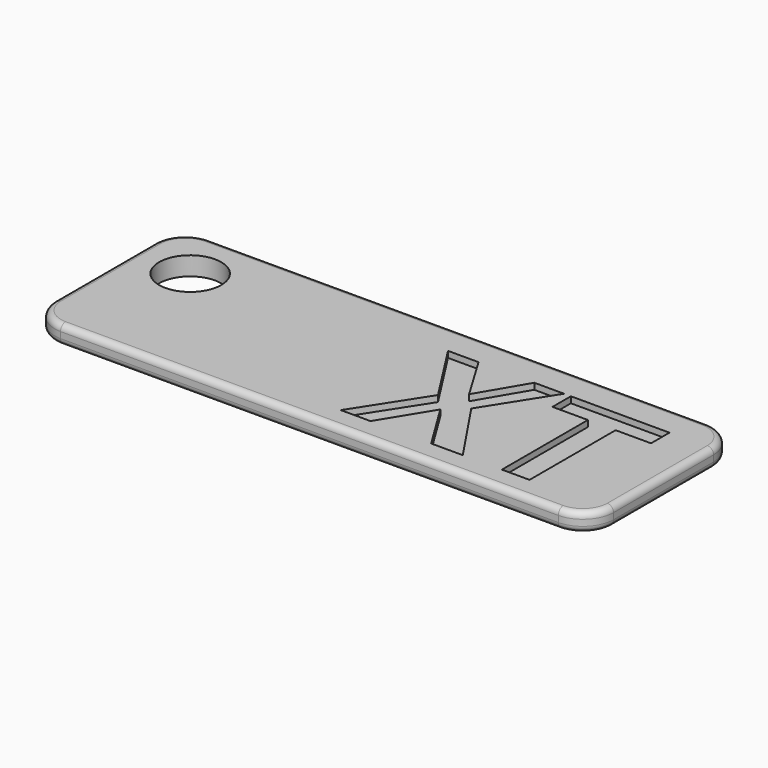
from build123d import *

# Parameters (mm, degrees)
F0_W         = 90
F0_H         = 30
F1_DEPTH     = 3
F2_R         = 1
F3_T3_ANGLE  = 90
F3_T6_ANGLE  = 90
F3_T9_ANGLE  = 90
F3_T12_ANGLE = 90
F3_T15_ANGLE = 90
F3_T18_ANGLE = 90
F3_T21_ANGLE = 90
F3_T24_ANGLE = 90
F3_T27_DEPTH = 3
F3_T30_DEPTH = 3
F3_T33_DEPTH = 3
F3_T36_DEPTH = 3
F4_R         = 5
F5_DEPTH     = 3
F6_TEXT_SIZE = 29.4359719196
F7_DEPTH     = 1


# Not quite as in the source:
# - a fillet or chamfer that OpenCascade refuses, or shapes differently, is made with other operations: its cross-section is extruded or revolved along the edge and cut away or added
# - Text() gives the source's letters only with a copy of the font that has no kerning and outlines rounded to 1/6400 em; it was checked with that copy


with BuildPart() as f1:
    # F0 (on Top) → F1 (new body)
    with BuildSketch(Plane.XY):
        Rectangle(F0_W, F0_H)
    extrude(amount=F1_DEPTH)

    # F2
    f2_edges = [f1.edges().sort_by_distance(p)[0] for p in [
        (0, 15, 3),
        (-45, 0, 3),
        (0, -15, 3),
        (45, 0, 3),
        (0, 15, 0),
        (-45, 0, 0),
        (0, -15, 0),
        (45, 0, 0),
    ]]
    fillet(f2_edges, radius=F2_R)

    # F3: fillet of radius 5 on 4 edges, made by hand


with BuildPart() as f3_tool1:
    # F3_s2 → F3_t3 (revolve)
    with BuildSketch(Plane.YZ.offset(-39.9990343146)):
        with BuildLine():
            ThreePointArc((-14.0004, 0), (-14.7075067812, 0.2928932188), (-15.0004, 1))
            Line((-15.0004, 1), (-15.0004, 0))
            Line((-15.0004, 0), (-14.0004, 0))
        make_face()
    revolve(axis=Axis((-39.9990343146, -9.9990343146, 0), (0, 0, -1)), revolution_arc=F3_T3_ANGLE)


with BuildPart() as f3_tool4:
    # F3_s5 → F3_t6 (revolve)
    with BuildSketch(Plane.XZ.offset(9.9990343146)):
        with BuildLine():
            ThreePointArc((-44.0004, 3), (-44.7075067812, 2.7071067812), (-45.0004, 2))
            Line((-45.0004, 2), (-45.0004, 3))
            Line((-45.0004, 3), (-44.0004, 3))
        make_face()
    revolve(axis=Axis((-39.9990343146, -9.9990343146, 3), (0, 0, 1)), revolution_arc=F3_T6_ANGLE)


with BuildPart() as f3_tool7:
    # F3_s8 → F3_t9 (revolve)
    with BuildSketch(Plane.XZ.offset(-9.9990343146)):
        with BuildLine():
            ThreePointArc((-44.0004, 0), (-44.7075067812, 0.2928932188), (-45.0004, 1))
            Line((-45.0004, 1), (-45.0004, 0))
            Line((-45.0004, 0), (-44.0004, 0))
        make_face()
    revolve(axis=Axis((-39.9990343146, 9.9990343146, 0), (0, 0, -1)), revolution_arc=F3_T9_ANGLE)


with BuildPart() as f3_tool10:
    # F3_s11 → F3_t12 (revolve)
    with BuildSketch(Plane.YZ.offset(-39.9990343146)):
        with BuildLine():
            ThreePointArc((14.0004, 3), (14.7075067812, 2.7071067812), (15.0004, 2))
            Line((15.0004, 2), (15.0004, 3))
            Line((15.0004, 3), (14.0004, 3))
        make_face()
    revolve(axis=Axis((-39.9990343146, 9.9990343146, 3), (0, 0, 1)), revolution_arc=F3_T12_ANGLE)


with BuildPart() as f3_tool13:
    # F3_s14 → F3_t15 (revolve)
    with BuildSketch(Plane.YZ.offset(39.9990343146)):
        with BuildLine():
            ThreePointArc((14.0004, 0), (14.7075067812, 0.2928932188), (15.0004, 1))
            Line((15.0004, 1), (15.0004, 0))
            Line((15.0004, 0), (14.0004, 0))
        make_face()
    revolve(axis=Axis((39.9990343146, 9.9990343146, 0), (0, 0, -1)), revolution_arc=F3_T15_ANGLE)


with BuildPart() as f3_tool16:
    # F3_s17 → F3_t18 (revolve)
    with BuildSketch(Plane.XZ.offset(-9.9990343146)):
        with BuildLine():
            ThreePointArc((44.0004, 3), (44.7075067812, 2.7071067812), (45.0004, 2))
            Line((45.0004, 2), (45.0004, 3))
            Line((45.0004, 3), (44.0004, 3))
        make_face()
    revolve(axis=Axis((39.9990343146, 9.9990343146, 3), (0, 0, 1)), revolution_arc=F3_T18_ANGLE)


with BuildPart() as f3_tool19:
    # F3_s20 → F3_t21 (revolve)
    with BuildSketch(Plane.XZ.offset(9.9990343146)):
        with BuildLine():
            ThreePointArc((44.0004, 0), (44.7075067812, 0.2928932188), (45.0004, 1))
            Line((45.0004, 1), (45.0004, 0))
            Line((45.0004, 0), (44.0004, 0))
        make_face()
    revolve(axis=Axis((39.9990343146, -9.9990343146, 0), (0, 0, -1)), revolution_arc=F3_T21_ANGLE)


with BuildPart() as f3_tool22:
    # F3_s23 → F3_t24 (revolve)
    with BuildSketch(Plane.YZ.offset(39.9990343146)):
        with BuildLine():
            ThreePointArc((-14.0004, 3), (-14.7075067812, 2.7071067812), (-15.0004, 2))
            Line((-15.0004, 2), (-15.0004, 3))
            Line((-15.0004, 3), (-14.0004, 3))
        make_face()
    revolve(axis=Axis((39.9990343146, -9.9990343146, 3), (0, 0, 1)), revolution_arc=F3_T24_ANGLE)


with BuildPart() as f3_tool25:
    # F3_s26 → F3_t27 (new body)
    with BuildSketch(Plane.XY):
        with BuildLine():
            ThreePointArc((45.0004, -9.9990343146), (43.5355339059, -13.5355339059), (39.9990343146, -15.0004))
            Line((39.9990343146, -15.0004), (39.9990343146, -15.5005365685))
            ThreePointArc((39.9990343146, -15.5005365685), (42.4995171573, -15.5001365685), (45, -15.5001365685))
            Line((45, -15.5001365685), (45.5001365685, -15))
            ThreePointArc((45.5001365685, -15), (45.5001365685, -12.4995171573), (45.5005365685, -9.9990343146))
            Line((45.5005365685, -9.9990343146), (45.0004, -9.9990343146))
        make_face()
    extrude(amount=F3_T27_DEPTH)


with BuildPart() as f3_tool28:
    # F3_s29 → F3_t30 (new body)
    with BuildSketch(Plane.XY):
        with BuildLine():
            ThreePointArc((39.9990343146, 15.0004), (43.5355339059, 13.5355339059), (45.0004, 9.9990343146))
            Line((45.0004, 9.9990343146), (45.5005365685, 9.9990343146))
            ThreePointArc((45.5005365685, 9.9990343146), (45.5001365685, 12.4995171573), (45.5001365685, 15))
            Line((45.5001365685, 15), (45, 15.5001365685))
            ThreePointArc((45, 15.5001365685), (42.4995171573, 15.5001365685), (39.9990343146, 15.5005365685))
            Line((39.9990343146, 15.5005365685), (39.9990343146, 15.0004))
        make_face()
    extrude(amount=F3_T30_DEPTH)


with BuildPart() as f3_tool31:
    # F3_s32 → F3_t33 (new body)
    with BuildSketch(Plane.XY):
        with BuildLine():
            ThreePointArc((-39.9990343146, 15.0004), (-43.5355339059, 13.5355339059), (-45.0004, 9.9990343146))
            Line((-45.0004, 9.9990343146), (-45.5005365685, 9.9990343146))
            ThreePointArc((-45.5005365685, 9.9990343146), (-45.5001365685, 12.4995171573), (-45.5001365685, 15))
            Line((-45.5001365685, 15), (-45, 15.5001365685))
            ThreePointArc((-45, 15.5001365685), (-42.4995171573, 15.5001365685), (-39.9990343146, 15.5005365685))
            Line((-39.9990343146, 15.5005365685), (-39.9990343146, 15.0004))
        make_face()
    extrude(amount=F3_T33_DEPTH)


with BuildPart() as f3_tool34:
    # F3_s35 → F3_t36 (new body)
    with BuildSketch(Plane.XY):
        with BuildLine():
            ThreePointArc((-45.0004, -9.9990343146), (-43.5355339059, -13.5355339059), (-39.9990343146, -15.0004))
            Line((-39.9990343146, -15.0004), (-39.9990343146, -15.5005365685))
            ThreePointArc((-39.9990343146, -15.5005365685), (-42.4995171573, -15.5001365685), (-45, -15.5001365685))
            Line((-45, -15.5001365685), (-45.5001365685, -15))
            ThreePointArc((-45.5001365685, -15), (-45.5001365685, -12.4995171573), (-45.5005365685, -9.9990343146))
            Line((-45.5005365685, -9.9990343146), (-45.0004, -9.9990343146))
        make_face()
    extrude(amount=F3_T36_DEPTH)


with BuildPart() as f1_1:
    add(f1.part)

    # F3_t37: cut F3_tool1, F3_tool4, F3_tool7, F3_tool10, F3_tool13, F3_tool16, F3_tool19, F3_tool22, F3_tool25, F3_tool28, F3_tool31, F3_tool34
    add([f3_tool1.part, f3_tool4.part, f3_tool7.part, f3_tool10.part, f3_tool13.part, f3_tool16.part, f3_tool19.part, f3_tool22.part, f3_tool25.part, f3_tool28.part, f3_tool31.part, f3_tool34.part], mode=Mode.SUBTRACT)

    # F4 (on face) → F5 (cut)
    with BuildSketch(Plane.XY.offset(3)):
        with Locations((-36, 6)):
            Circle(F4_R)
    extrude(amount=-F5_DEPTH, mode=Mode.SUBTRACT)

    # F6 (on face) → F7 (cut)
    with BuildSketch(Plane.XY.offset(3)):
        with Locations((2, -11.1938997821)):
            Text('XT', F6_TEXT_SIZE, font='Open Sans', font_style=FontStyle.BOLD, text_align=(TextAlign.LEFT, TextAlign.BOTTOM))
    extrude(amount=-F7_DEPTH, mode=Mode.SUBTRACT)


solid = f1_1.part
